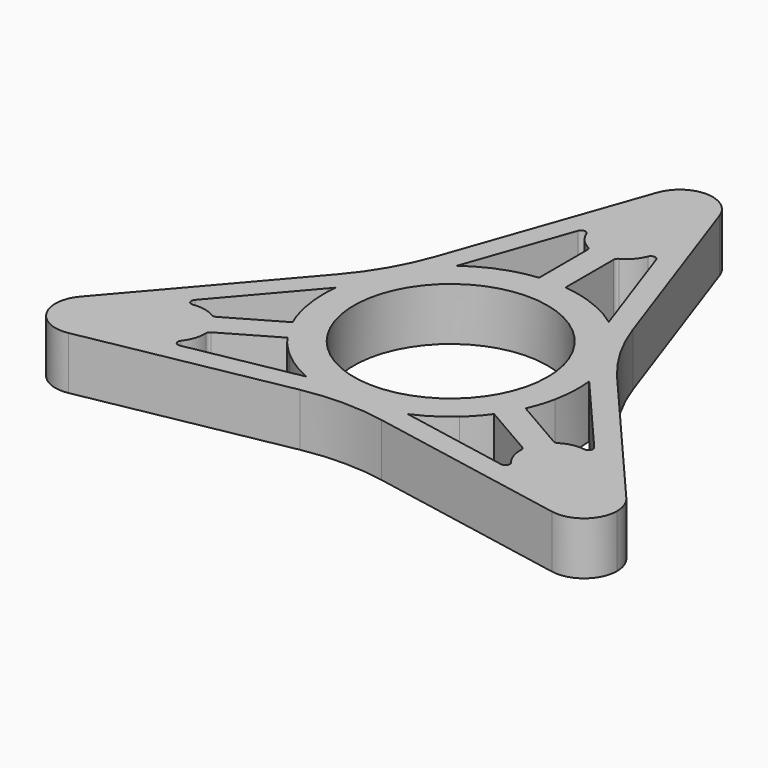
from build123d import *

# Parameters (mm, degrees)
F0_R     = 11
F1_DEPTH = 6


# Not quite as in the source:
# - a feature names something its author has since deleted; it is built from what else it names


with BuildPart() as f1:
    # F0 (on Top) → F1 (new body)
    with BuildSketch(Plane.XY):
        with BuildLine():
            Line((-17.653754974, -11.924450994), (-11.7399959968, -8.5101406566))
            ThreePointArc((-11.7399959968, -8.5101406566), (-10.7595852813, -9.7201504399), (-9.655057883, -10.8180338914))
            ThreePointArc((-9.655057883, -10.8180338914), (-7.8135298696, -12.2146940599), (-5.7734811503, -13.3010118189))
            Line((-5.7734811503, -13.3010118189), (-18.2459966778, -15.6542301338))
            ThreePointArc((-18.2459966778, -15.6542301338), (-18.7675177207, -15.4200232887), (-18.72842119, -14.8496650628))
            ThreePointArc((-18.72842119, -14.8496650628), (-21.1687491133, -16.2192293875), (-23.8778204631, -15.5179168796))
            ThreePointArc((-23.8778204631, -15.5179168796), (-24.4287426612, -15.0200539994), (-24.8707648644, -14.4233974084))
            ThreePointArc((-24.8707648644, -14.4233974084), (-24.516502143, -15.306331055), (-24.395825623, -16.25))
            ThreePointArc((-24.395825623, -16.25), (-25.2588111204, -18.643250355), (-27.4505708292, -19.9349858577))
            Line((-27.4505708292, -19.9349858577), (-4.6350319583, -15.6303254372))
            ThreePointArc((-4.6350319583, -15.6303254372), (0, -15.1968978222), (4.6350319583, -15.6303254372))
            Line((4.6350319583, -15.6303254372), (27.4505708292, -19.9349858577))
            ThreePointArc((27.4505708292, -19.9349858577), (24.7494668073, -17.8397316739), (24.8707648644, -14.4233974084))
            ThreePointArc((24.8707648644, -14.4233974084), (27.7689882832, -12.5189822274), (30.9894895915, -13.8053987576))
            Line((30.9894895915, -13.8053987576), (15.8537748772, 3.8011072954))
            ThreePointArc((15.8537748772, 3.8011072954), (13.1608995727, 7.5984489111), (11.2187429189, 11.8292181419))
            Line((11.2187429189, 11.8292181419), (3.5389187623, 33.7403846154))
            ThreePointArc((3.5389187623, 33.7403846154), (0, 36.25), (-3.5389187623, 33.7403846154))
            Line((-3.5389187623, 33.7403846154), (-11.2187429189, 11.8292181419))
            ThreePointArc((-11.2187429189, 11.8292181419), (-13.1608995727, 7.5984489111), (-15.8537748772, 3.8011072954))
            Line((-15.8537748772, 3.8011072954), (-30.9894895915, -13.8053987576))
            ThreePointArc((-30.9894895915, -13.8053987576), (-27.8243942299, -12.5138011483), (-24.9264109967, -14.32701548))
            ThreePointArc((-24.9264109967, -14.32701548), (-25.2221196603, -13.6458847274), (-25.3778204631, -12.9198406683))
            ThreePointArc((-25.3778204631, -12.9198406683), (-24.630639236, -10.2230598047), (-22.2243977771, -8.7944559919))
            ThreePointArc((-22.2243977771, -8.7944559919), (-22.7378907553, -8.5431354678), (-22.6799593114, -7.9743815734))
            Line((-22.6799593114, -7.9743815734), (-14.4057547064, 1.650524565))
            ThreePointArc((-14.4057547064, 1.650524565), (-14.4569527647, -0.6438963434), (-14.1689115613, -2.9207408288))
            ThreePointArc((-14.1689115613, -2.9207408288), (-13.7801833851, -4.4399194539), (-13.2399959968, -5.9120644453))
            Line((-13.2399959968, -5.9120644453), (-19.153754974, -9.3263747827))
            ThreePointArc((-19.153754974, -9.3263747827), (-19.4121649397, -9.3932913482), (-19.6681779463, -9.3177209993))
            ThreePointArc((-19.6681779463, -9.3177209993), (-18.403754974, -10.6254128883), (-17.9034720639, -12.374281248))
            ThreePointArc((-17.9034720639, -12.374281248), (-17.8409114026, -12.1147823061), (-17.653754974, -11.924450994))
        make_face()
        with BuildLine():
            ThreePointArc((17.9034720639, -12.374281248), (18.093710781, -13.6860357173), (18.72842119, -14.8496650628))
            ThreePointArc((18.72842119, -14.8496650628), (18.7675177207, -15.4200232887), (18.2459966778, -15.6542301338))
            Line((18.2459966778, -15.6542301338), (5.7734811503, -13.3010118189))
            ThreePointArc((5.7734811503, -13.3010118189), (7.8135298696, -12.2146940599), (9.655057883, -10.8180338914))
            ThreePointArc((9.655057883, -10.8180338914), (10.7595852813, -9.7201504399), (11.7399959968, -8.5101406566))
            Line((11.7399959968, -8.5101406566), (17.653754974, -11.924450994))
            ThreePointArc((17.653754974, -11.924450994), (17.8409114026, -12.1147823061), (17.9034720639, -12.374281248))
        make_face(mode=Mode.SUBTRACT)
        Circle(F0_R, mode=Mode.SUBTRACT)
        with BuildLine():
            ThreePointArc((22.2243977771, -8.7944559919), (20.8993099987, -8.8265953264), (19.6681779463, -9.3177209993))
            ThreePointArc((19.6681779463, -9.3177209993), (19.4121649397, -9.3932913482), (19.153754974, -9.3263747827))
            Line((19.153754974, -9.3263747827), (13.2399959968, -5.9120644453))
            ThreePointArc((13.2399959968, -5.9120644453), (13.7976898502, -4.4579989679), (14.1962211105, -2.952508456))
            ThreePointArc((14.1962211105, -2.952508456), (14.4850002901, -0.6593683303), (14.4057547064, 1.650524565))
            Line((14.4057547064, 1.650524565), (22.6799593114, -7.9743815734))
            ThreePointArc((22.6799593114, -7.9743815734), (22.7378907553, -8.5431354678), (22.2243977771, -8.7944559919))
        make_face(mode=Mode.SUBTRACT)
        with BuildLine():
            ThreePointArc((-3.4959765871, 23.6441210547), (-2.8055992178, 22.5126310437), (-1.7647058824, 21.6920022473))
            ThreePointArc((-1.7647058824, 21.6920022473), (-1.5712535371, 21.5080736544), (-1.5, 21.2508257767))
            Line((-1.5, 21.2508257767), (-1.5, 14.4222051019))
            ThreePointArc((-1.5, 14.4222051019), (-3.0381045689, 14.1781494077), (-4.5411632274, 13.7705423474))
            ThreePointArc((-4.5411632274, 13.7705423474), (-6.6714704205, 12.8740623902), (-8.632273556, 11.6504872539))
            Line((-8.632273556, 11.6504872539), (-4.4339626337, 23.6286117072))
            ThreePointArc((-4.4339626337, 23.6286117072), (-3.9703730346, 23.9631587565), (-3.4959765871, 23.6441210547))
        make_face(mode=Mode.SUBTRACT)
        with BuildLine():
            ThreePointArc((3.4959765871, 23.6441210547), (3.9703730346, 23.9631587565), (4.4339626337, 23.6286117072))
            Line((4.4339626337, 23.6286117072), (8.632273556, 11.6504872539))
            ThreePointArc((8.632273556, 11.6504872539), (6.6711103348, 12.8576010839), (4.5482718222, 13.7502609452))
            ThreePointArc((4.5482718222, 13.7502609452), (3.041663637, 14.1657474781), (1.5, 14.4222051019))
            Line((1.5, 14.4222051019), (1.5, 21.2508257767))
            ThreePointArc((1.5, 21.2508257767), (1.5712535371, 21.5080736544), (1.7647058824, 21.6920022473))
            ThreePointArc((1.7647058824, 21.6920022473), (2.8055992178, 22.5126310437), (3.4959765871, 23.6441210547))
        make_face(mode=Mode.SUBTRACT)
        with BuildLine():
            ThreePointArc((-18.72842119, -14.8496650628), (-18.093710781, -13.6860357173), (-17.9034720639, -12.374281248))
            ThreePointArc((-17.9034720639, -12.374281248), (-18.403754974, -10.6254128883), (-19.6681779463, -9.3177209993))
            ThreePointArc((-19.6681779463, -9.3177209993), (-20.8993099987, -8.8265953264), (-22.2243977771, -8.7944559919))
            ThreePointArc((-22.2243977771, -8.7944559919), (-24.630639236, -10.2230598047), (-25.3778204631, -12.9198406683))
            ThreePointArc((-25.3778204631, -12.9198406683), (-25.2221196603, -13.6458847274), (-24.9264109967, -14.32701548))
            ThreePointArc((-24.9264109967, -14.32701548), (-24.8982303588, -14.375), (-24.8707648644, -14.4233974084))
            ThreePointArc((-24.8707648644, -14.4233974084), (-24.4287426612, -15.0200539994), (-23.8778204631, -15.5179168796))
            ThreePointArc((-23.8778204631, -15.5179168796), (-21.1687491133, -16.2192293875), (-18.72842119, -14.8496650628))
        make_face()
        with BuildLine():
            ThreePointArc((-24.395825623, -16.25), (-24.516502143, -15.306331055), (-24.8707648644, -14.4233974084))
            ThreePointArc((-24.8707648644, -14.4233974084), (-24.8982303588, -14.375), (-24.9264109967, -14.32701548))
            ThreePointArc((-24.9264109967, -14.32701548), (-27.8243942299, -12.5138011483), (-30.9894895915, -13.8053987576))
            ThreePointArc((-30.9894895915, -13.8053987576), (-31.3934208872, -18.125), (-27.4505708292, -19.9349858577))
            ThreePointArc((-27.4505708292, -19.9349858577), (-25.2588111204, -18.643250355), (-24.395825623, -16.25))
        make_face()
        with BuildLine():
            ThreePointArc((24.8707648644, -14.4233974084), (24.7494668073, -17.8397316739), (27.4505708292, -19.9349858577))
            ThreePointArc((27.4505708292, -19.9349858577), (30.539075978, -19.1370145026), (31.895825623, -16.25))
            ThreePointArc((31.895825623, -16.25), (31.6619484793, -14.9463972771), (30.9894895915, -13.8053987576))
            ThreePointArc((30.9894895915, -13.8053987576), (27.7689882832, -12.5189822274), (24.8707648644, -14.4233974084))
        make_face()
    extrude(amount=F1_DEPTH)


solid = f1.part
